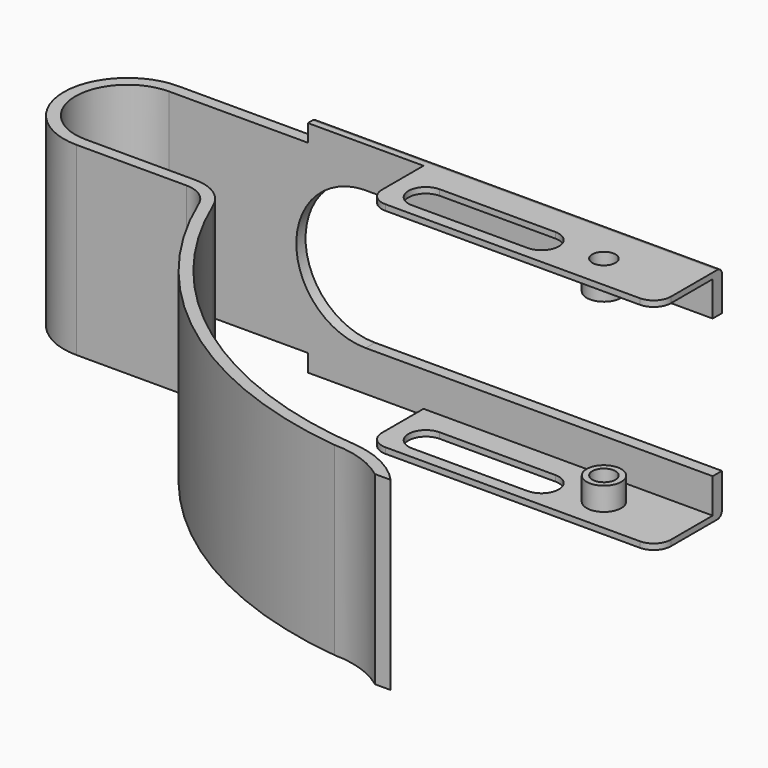
from build123d import *

# Parameters (mm, degrees)
F1_DEPTH  = 16
F2_W      = 70
F2_H      = 3
F3_DEPTH  = 2
F4_W      = 50
F4_H      = 14
F5_DEPTH  = 1
F6_R      = 1
F9_DEPTH  = 2
F11_DEPTH = 1.001
F13_D     = 4
F13_DEPTH = 50
F13_TIP   = 1.2017212381
F14_R     = 3
F14_R_2   = 2
F15_DEPTH = 5
F16_R     = 3
F18_D     = 4
F18_DEPTH = 50
F18_TIP   = 1.2017212381


# Not quite as in the source:
# - a pattern or mirror of a feature is missing from the dataset's text; its kind, count and spacing are read off the source's solid


with BuildPart() as f1:
    # F0 (on Top) → F1 (new body)
    with BuildSketch(Plane.XY):
        with BuildLine():
            Line((94, 11), (0, 11))
            ThreePointArc((0, 11), (-11, 0), (0, -11))
            Line((0, -11), (19, -11))
            ThreePointArc((19, -11), (21.7681124643, -11.8361612201), (23.6103896104, -14.064978646))
            ThreePointArc((23.6103896104, -14.064978646), (46.8644288503, -43.8489365308), (81.9993431207, -57.7547729841))
            ThreePointArc((81.9993431207, -57.7547729841), (87.0632727772, -58.5972193444), (91.5997631119, -61))
            Line((91.5997631119, -61), (94.3248553538, -61))
            ThreePointArc((94.3248553538, -61), (89.9506080698, -57.6601123846), (84.7034264019, -56))
            ThreePointArc((84.7034264019, -56), (49.0672193413, -42.9854179344), (25.4545454545, -13.2909701044))
            ThreePointArc((25.4545454545, -13.2909701044), (22.87535745, -10.1706257081), (19, -9))
            Line((19, -9), (0, -9))
            ThreePointArc((0, -9), (-9, 0), (0, 9))
            Line((0, 9), (94, 9))
            Line((94, 9), (94, 11))
        make_face()
    extrude(amount=F1_DEPTH)

    # F2 (on face) → F3 (join)
    with BuildSketch(Plane(origin=(0, 11, 0), x_dir=(-1, 0, 0), z_dir=(0, 1, 0))):
        with Locations((-59, 17.5)):
            Rectangle(F2_W, F2_H)
    extrude(amount=-F3_DEPTH)

    # F4 (on face) → F5 (join)
    with BuildSketch(Plane.XY.offset(19)):
        with Locations((69, 4)):
            Rectangle(F4_W, F4_H)
    extrude(amount=-F5_DEPTH)

    # F6
    f6_edges = [f1.edges().sort_by_distance(p)[0] for p in [
        (59, 11, 19),
    ]]
    fillet(f6_edges, radius=F6_R)

    # F7: F1 across face


with BuildPart() as f1_1:
    add(f1.part)
    add(f1.part.mirror(Plane(origin=(39.0198924269, -12.8147332924, 0), x_dir=(1, 0, 0), z_dir=(0, 0, -1))))

    # F8 (on face) → F9 (cut)
    with BuildSketch(Plane(origin=(0, 11, 0), x_dir=(-1, 0, 0), z_dir=(0, 1, 0))):
        with BuildLine():
            Line((-94, -12), (-34, -12))
            ThreePointArc((-34, -12), (-22.001130085, -0.1646838272), (-33.6706633635, 11.9954798728))
            Line((-33.6706633635, 11.9954798728), (-34.3293366365, 11.9954798728))
            Line((-34.3293366365, 11.9954798728), (-94, 11.9954798728))
            Line((-94, 11.9954798728), (-94, -12))
        make_face()
    extrude(amount=-F9_DEPTH, mode=Mode.SUBTRACT)

    # F10 (on face) → F11 (cut, through all)
    with BuildSketch(Plane(origin=(0, 0, 18), x_dir=(1, 0, 0), z_dir=(0, 0, -1))):
        with BuildLine():
            ThreePointArc((50, 1), (47, -2), (50, -5))
            Line((50, -5), (70, -5))
            ThreePointArc((70, -5), (73, -2), (70, 1))
            Line((70, 1), (50, 1))
        make_face()
    f11 = extrude(amount=-F11_DEPTH, mode=Mode.SUBTRACT)

    # F11_copies: F11 across plane
    add(f11.mirror(Plane(origin=(0, 0, 0), x_dir=(-1, 0, 0), z_dir=(0, 0, -1))), mode=Mode.SUBTRACT)

    # F13 (one way)
    with BuildSketch(Plane.XY.offset(18)):
        with Locations((80, 3)):
            Circle(F13_D / 2)
    extrude(amount=-F13_DEPTH, mode=Mode.SUBTRACT)
    with Locations(Plane.XY.offset(18)):
        with Locations((80, 3)):
            with Locations((0, 0, -(F13_DEPTH + F13_TIP / 2))):  # 118° drill point
                Cone(0, F13_D / 2, F13_TIP, mode=Mode.SUBTRACT)

    # F14 (on face) → F15 (join)
    with BuildSketch(Plane.XY.offset(19)):
        with Locations((80, 3)):
            Circle(F14_R)
        with Locations((80, 3)):
            Circle(F14_R_2, mode=Mode.SUBTRACT)
    f15 = extrude(amount=-F15_DEPTH)

    # F15_copies: F15 across plane
    add(f15.mirror(Plane(origin=(0, 0, 0), x_dir=(-1, 0, 0), z_dir=(0, 0, -1))))

    # F16
    f16_edges = [f1_1.edges().sort_by_distance(p)[0] for p in [
        (94, -3, 18.5),
        (44, -3, 18.5),
        (44, -3, -18.5),
        (94, -3, -18.5),
    ]]
    fillet(f16_edges, radius=F16_R)

    # F18
    with Locations(Plane.XY.offset(19)):
        with Locations((79.9801871181, 3.0164394993)):
            Hole(F18_D / 2, depth=F18_DEPTH)
            with Locations((0, 0, -(F18_DEPTH + F18_TIP / 2))):  # 118° drill point
                Cone(0, F18_D / 2, F18_TIP, mode=Mode.SUBTRACT)


solid = f1_1.part
